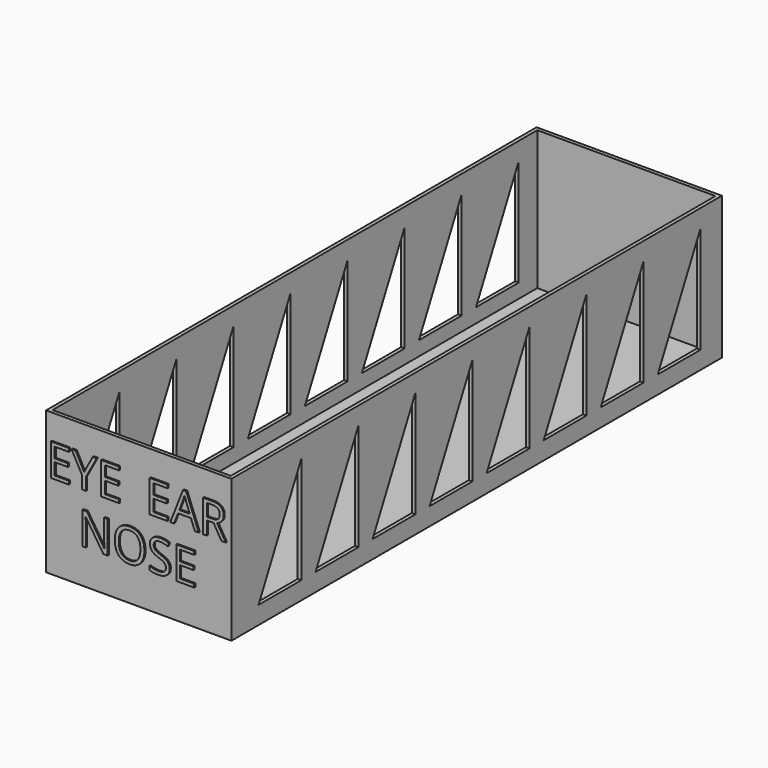
from build123d import *

# Parameters (mm, degrees)
F0_W         = 66.04
F0_H         = 218.44
F0_W_2       = 63.5
F0_H_2       = 215.9
F1_DEPTH     = 1.27
F2_DEPTH     = 50.8
F4_DEPTH     = 76.2
F5_TEXT_SIZE = 16.0513888889
F6_DEPTH     = 0.508


# Not quite as in the source:
# - Text() gives the source's letters only with a copy of the font that has no kerning and outlines rounded to 1/6400 em; it was checked with that copy


with BuildPart() as f1:
    # F0 (on Top) → F1 (new body)
    with BuildSketch(Plane.XY):
        Rectangle(F0_W, F0_H)
        Rectangle(F0_W_2, F0_H_2, mode=Mode.SUBTRACT)
        Rectangle(F0_W_2, F0_H_2)
    extrude(amount=F1_DEPTH)

    # F0 (on Top) → F2 (join)
    with BuildSketch(Plane.XY):
        Rectangle(F0_W, F0_H)
        Rectangle(F0_W_2, F0_H_2, mode=Mode.SUBTRACT)
    extrude(amount=F2_DEPTH)

    # F3 (on face) → F4 (cut)
    with BuildSketch(Plane(origin=(-33.02, 0, 0), x_dir=(0, -1, 0), z_dir=(-1, 0, 0))):
        Polygon((-80.645, 6.35), (-99.695, 44.45), (-99.695, 6.35), align=None)
        Polygon((-74.295, 6.35), (-55.245, 6.35), (-74.295, 44.45), align=None)
        Polygon((-48.895, 6.35), (-29.845, 6.35), (-48.895, 44.45), align=None)
        Polygon((-23.495, 6.35), (-4.445, 6.35), (-23.495, 44.45), align=None)
        Polygon((1.905, 6.35), (20.955, 6.35), (1.905, 44.45), align=None)
        Polygon((27.305, 6.35), (46.355, 6.35), (27.305, 44.45), align=None)
        Polygon((52.705, 6.35), (71.755, 6.35), (52.705, 44.45), align=None)
        Polygon((78.105, 6.35), (97.155, 6.35), (78.105, 44.45), align=None)
    extrude(amount=-F4_DEPTH, mode=Mode.SUBTRACT)

    # F5 (on face) → F6 (join)
    with BuildSketch(Plane.XZ.offset(109.22)):
        with Locations((-32.4777281901, 30.48)):
            Text('EYE  EAR', F5_TEXT_SIZE, font='Open Sans', text_align=(TextAlign.LEFT, TextAlign.BOTTOM))
        with Locations((-21.2078975694, 12.7)):
            Text('NOSE', F5_TEXT_SIZE, font='Open Sans', text_align=(TextAlign.LEFT, TextAlign.BOTTOM))
    extrude(amount=F6_DEPTH)


solid = f1.part
